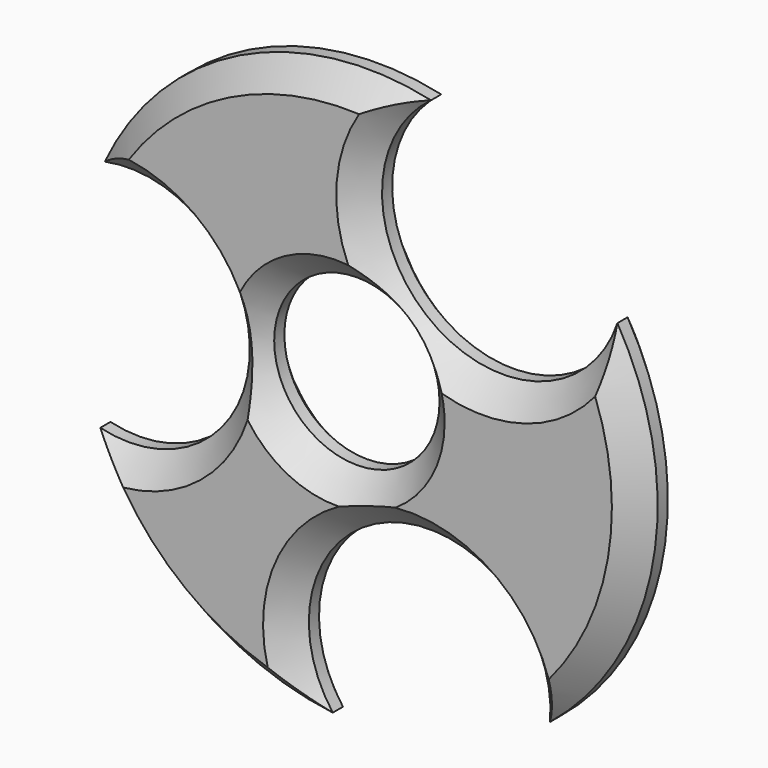
from build123d import *

# Parameters (mm, degrees)
F0_R         = 57.9360533335
F2_DEPTH     = 12.7
F3_D         = 48.26
F5_D         = 33.02
F6_T2_ANGLE  = 283.4727948919
F6_T4_ANGLE  = 86.0712547595
F6_T6_ANGLE  = 107.4118170834
F6_T8_ANGLE  = 267.462303274
F6_T10_ANGLE = 277.2145700269
F6_T12_ANGLE = 103.4165555336
F6_T16_ANGLE = 107.4118170834
F6_T18_ANGLE = 283.4727948919
F6_T20_ANGLE = 277.2145700269
F6_T22_ANGLE = 86.0712547595
F6_T24_ANGLE = 103.4165555336
F6_T26_ANGLE = 267.462303274


# Not quite as in the source:
# - a fillet or chamfer that OpenCascade refuses, or shapes differently, is made with other operations: its cross-section is extruded or revolved along the edge and cut away or added


with BuildPart() as f2:
    # F0 (on Front) → F2 (new body)
    with BuildSketch(Plane.XZ):
        with Locations((-72.7998018265, -8.9674890041)):
            Circle(F0_R)
    extrude(amount=F2_DEPTH)

    # F3 (through all)
    with Locations(Plane(origin=(0, 0, 0), x_dir=(1, 0, 0), z_dir=(0, 1, 0))):
        with Locations((-45.7866154611, -28.1515028328), (-120.4445809126, 8.0565353855), (-60.4006908834, 52.0677864552)):
            Hole(F3_D / 2)

    # F5 (through all)
    with Locations(Plane(origin=(0, 0, 0), x_dir=(1, 0, 0), z_dir=(0, 1, 0))):
        with Locations((-74.9381706119, 4.8889117315)):
            Hole(F5_D / 2)

    # F6: chamfer of 5.08 on 14 edges, made by hand

    # F6_s1 → F6_t2 (revolve, cut)
    with BuildSketch(Plane(origin=(-33.5431340109, 0, 13.6983383479), x_dir=(0, 1, 0), z_dir=(0.9257774909, 0, -0.3780688263))):
        Polygon((-7.62, -95.1688030077), (-12.7, -100.2488030077), (-12.7, -95.1688030077), align=None)
    revolve(axis=Axis((-60.4006908834, -12.7, -52.0677864552), (0, 1, 0)), revolution_arc=F6_T2_ANGLE, mode=Mode.SUBTRACT)

    # F6_s3 → F6_t4 (revolve, cut)
    with BuildSketch(Plane(origin=(-0.6504253771, 0, 3.7035474889), x_dir=(0, 1, 0), z_dir=(-0.1729749681, 0, 0.9849262208))):
        Polygon((-12.7, 126.1096381457), (-7.62, 131.1896381457), (-12.7, 131.1896381457), align=None)
    revolve(axis=Axis((-72.7998018265, -12.7, -8.9674890041), (0, -1, 0)), revolution_arc=F6_T4_ANGLE, mode=Mode.SUBTRACT)

    # F6_s5 → F6_t6 (revolve, cut)
    with BuildSketch(Plane(origin=(-29.9879926822, 0, 31.6264228209), x_dir=(0, 1, 0), z_dir=(-0.6880604052, 0, 0.7256534151))):
        Polygon((-7.62, 1.0615455961), (-12.7, 6.1415455961), (-12.7, 1.0615455961), align=None)
    revolve(axis=Axis((-72.7998018265, -12.7, -8.9674890041), (0, 1, 0)), revolution_arc=F6_T6_ANGLE, mode=Mode.SUBTRACT)

    # F6_s7 → F6_t8 (revolve, cut)
    with BuildSketch(Plane(origin=(-69.201107614, 0, -63.7135426846), x_dir=(0, 1, 0), z_dir=(-0.7356739262, 0, -0.6773358652))):
        Polygon((-12.7, -104.8644514037), (-7.62, -99.7844514037), (-12.7, -99.7844514037), align=None)
    revolve(axis=Axis((-120.4445809126, -12.7, -8.0565353855), (0, 1, 0)), revolution_arc=F6_T8_ANGLE, mode=Mode.SUBTRACT)

    # F6_s9 → F6_t10 (revolve, cut)
    with BuildSketch(Plane(origin=(-8.1423267798, 0, 36.5399201696), x_dir=(0, 1, 0), z_dir=(-0.2174992035, 0, 0.9760604984))):
        Polygon((-12.7, 9.3575772605), (-7.62, 14.4375772605), (-12.7, 14.4375772605), align=None)
    revolve(axis=Axis((-45.7866154611, -12.7, 28.1515028328), (0, 1, 0)), revolution_arc=F6_T10_ANGLE, mode=Mode.SUBTRACT)

    # F6_s11 → F6_t12 (revolve, cut)
    with BuildSketch(Plane(origin=(-55.7502574842, 0, 26.6710376642), x_dir=(0, 1, 0), z_dir=(0.9020846433, 0, -0.4315591458))):
        Polygon((-12.7, 13.3491989235), (-7.62, 18.4291989235), (-12.7, 18.4291989235), align=None)
    revolve(axis=Axis((-72.7998018265, -12.7, -8.9674890041), (0, -1, 0)), revolution_arc=F6_T12_ANGLE, mode=Mode.SUBTRACT)

    # F6_s13 → F6_t14 (revolve, cut)
    with BuildSketch(Plane.XY.offset(-4.8889117315)):
        Polygon((-53.3481706119, -12.7), (-58.4281706119, -7.62), (-58.4281706119, -12.7), align=None)
    revolve(axis=Axis((-74.9381706119, -12.7, -4.8889117315), (0, 1, 0)), mode=Mode.SUBTRACT)

    # F6_s15 → F6_t16 (revolve, cut)
    with BuildSketch(Plane(origin=(-62.2843162467, 0, -30.4655418629), x_dir=(0, 1, 0), z_dir=(-0.8982965238, 0, -0.4393897533))):
        Polygon((-5.08, 34.004030567), (0, 28.924030567), (0, 34.004030567), align=None)
    revolve(axis=Axis((-72.7998018265, 0, -8.9674890041), (0, -1, 0)), revolution_arc=F6_T16_ANGLE, mode=Mode.SUBTRACT)

    # F6_s17 → F6_t18 (revolve, cut)
    with BuildSketch(Plane(origin=(-45.2248879791, 0, -62.9674495541), x_dir=(0, 1, 0), z_dir=(-0.5833556277, 0, -0.8122168501))):
        Polygon((0, 10.5255773581), (-5.08, 5.4455773581), (0, 5.4455773581), align=None)
    revolve(axis=Axis((-60.4006908834, 0, -52.0677864552), (0, -1, 0)), revolution_arc=F6_T18_ANGLE, mode=Mode.SUBTRACT)

    # F6_s19 → F6_t20 (revolve, cut)
    with BuildSketch(Plane(origin=(-8.1423267798, 0, 36.5399201696), x_dir=(0, 1, 0), z_dir=(-0.2174992035, 0, 0.9760604984))):
        Polygon((0, 9.3575772605), (-5.08, 14.4375772605), (0, 14.4375772605), align=None)
    revolve(axis=Axis((-45.7866154611, 0, 28.1515028328), (0, 1, 0)), revolution_arc=F6_T20_ANGLE, mode=Mode.SUBTRACT)

    # F6_s21 → F6_t22 (revolve, cut)
    with BuildSketch(Plane(origin=(-0.6504253771, 0, 3.7035474889), x_dir=(0, 1, 0), z_dir=(-0.1729749681, 0, 0.9849262208))):
        Polygon((0, 126.1096381457), (-5.08, 131.1896381457), (0, 131.1896381457), align=None)
    revolve(axis=Axis((-72.7998018265, 0, -8.9674890041), (0, -1, 0)), revolution_arc=F6_T22_ANGLE, mode=Mode.SUBTRACT)

    # F6_s23 → F6_t24 (revolve, cut)
    with BuildSketch(Plane(origin=(-55.7502574842, 0, 26.6710376642), x_dir=(0, 1, 0), z_dir=(0.9020846433, 0, -0.4315591458))):
        Polygon((0, 13.3491989235), (-5.08, 18.4291989235), (0, 18.4291989235), align=None)
    revolve(axis=Axis((-72.7998018265, 0, -8.9674890041), (0, -1, 0)), revolution_arc=F6_T24_ANGLE, mode=Mode.SUBTRACT)

    # F6_s25 → F6_t26 (revolve, cut)
    with BuildSketch(Plane(origin=(-56.5588266789, 0, 56.2173150628), x_dir=(0, 1, 0), z_dir=(-0.7092448082, 0, 0.7049622699))):
        Polygon((0, 119.832941055), (-5.08, 114.752941055), (0, 114.752941055), align=None)
    revolve(axis=Axis((-120.4445809126, 0, -8.0565353855), (0, -1, 0)), revolution_arc=F6_T26_ANGLE, mode=Mode.SUBTRACT)

    # F6_s27 → F6_t28 (revolve, cut)
    with BuildSketch(Plane.XY.offset(-4.8889117315)):
        Polygon((-53.3481706119, 0), (-58.4281706119, -5.08), (-58.4281706119, 0), align=None)
    revolve(axis=Axis((-74.9381706119, 0, -4.8889117315), (0, 1, 0)), mode=Mode.SUBTRACT)


solid = f2.part
